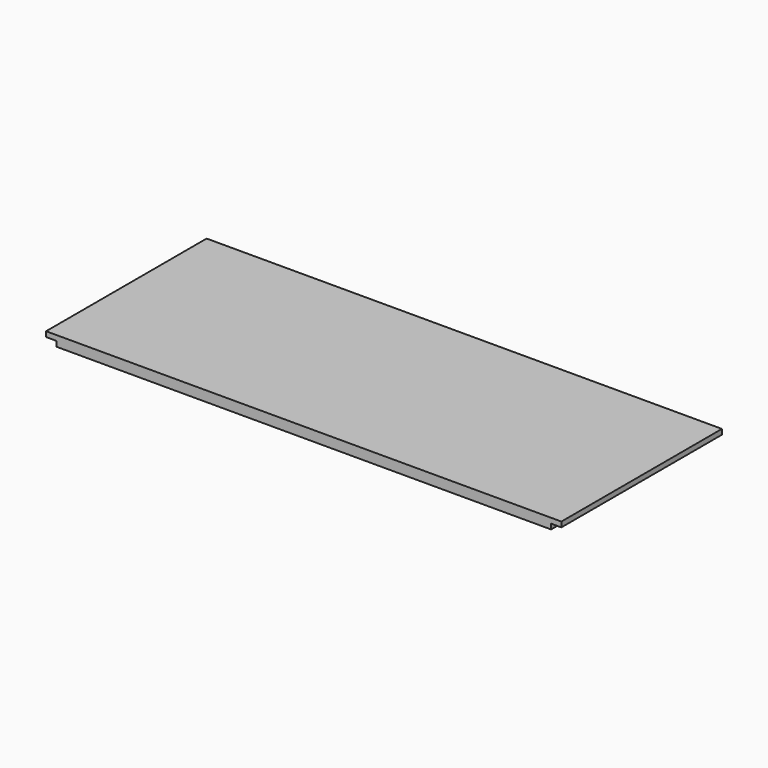
from build123d import *

# Parameters (mm, degrees)
F1_W      = 603.25
F1_H      = 234.95
F2_DEPTH  = 12.065
F3_W      = 12.065
F3_H      = 234.95
F4_DEPTH  = 6.0325
F5_W      = 12.065
F5_H      = 234.95
F6_DEPTH  = 6.0325
F7_W      = 12.065
F7_H      = 234.95
F8_DEPTH  = 6.0325
F9_W      = 12.065
F9_H      = 234.95
F10_DEPTH = 6.0325
F11_W     = 203.2
F11_H     = 12.065
F14_DEPTH = 6.0325
F12_W     = 148.59
F12_H     = 12.065
F15_DEPTH = 6.0325
F13_W     = 203.2
F13_H     = 12.065
F16_DEPTH = 6.0325
F17_W     = 12.065
F17_H     = 31.75
F18_DEPTH = 6.0325
F19_W     = 12.065
F19_H     = 31.75
F20_DEPTH = 6.0325


# Not quite as in the source:
# - a variable given as a bare number and used for a length is read in inches; the dataset says mm whatever the document's units were


with BuildPart() as f2:
    # F1 (on Top) → F2 (new body)
    with BuildSketch(Plane.XY):
        Rectangle(F1_W, F1_H)
    extrude(amount=F2_DEPTH)

    # F3 (on face) → F4 (cut)
    with BuildSketch(Plane(origin=(0, 0, 0), x_dir=(1, 0, 0), z_dir=(0, 0, -1))):
        with Locations((-295.5925, 0)):
            Rectangle(F3_W, F3_H)
    extrude(amount=-F4_DEPTH, mode=Mode.SUBTRACT)

    # F5 (on face) → F6 (cut)
    with BuildSketch(Plane(origin=(0, 0, 0), x_dir=(1, 0, 0), z_dir=(0, 0, -1))):
        with Locations((295.5925, 0)):
            Rectangle(F5_W, F5_H)
    extrude(amount=-F6_DEPTH, mode=Mode.SUBTRACT)

    # F7 (on face) → F8 (cut)
    with BuildSketch(Plane(origin=(0, 0, 0), x_dir=(1, 0, 0), z_dir=(0, 0, -1))):
        with Locations((80.3275, 0)):
            Rectangle(F7_W, F7_H)
    extrude(amount=-F8_DEPTH, mode=Mode.SUBTRACT)

    # F9 (on face) → F10 (cut)
    with BuildSketch(Plane(origin=(0, 0, 0), x_dir=(1, 0, 0), z_dir=(0, 0, -1))):
        with Locations((-80.3275, 0)):
            Rectangle(F9_W, F9_H)
    extrude(amount=-F10_DEPTH, mode=Mode.SUBTRACT)

    # F11 (on face) → F14 (cut)
    with BuildSketch(Plane(origin=(0, 0, 0), x_dir=(1, 0, 0), z_dir=(0, 0, -1))):
        with Locations((187.96, -111.4425)):
            Rectangle(F11_W, F11_H)
    extrude(amount=-F14_DEPTH, mode=Mode.SUBTRACT)

    # F12 (on face) → F15 (cut)
    with BuildSketch(Plane(origin=(0, 0, 0), x_dir=(1, 0, 0), z_dir=(0, 0, -1))):
        with Locations((0, -111.4425)):
            Rectangle(F12_W, F12_H)
    extrude(amount=-F15_DEPTH, mode=Mode.SUBTRACT)

    # F13 (on face) → F16 (cut)
    with BuildSketch(Plane(origin=(0, 0, 0), x_dir=(1, 0, 0), z_dir=(0, 0, -1))):
        with Locations((-187.96, -111.4425)):
            Rectangle(F13_W, F13_H)
    extrude(amount=-F16_DEPTH, mode=Mode.SUBTRACT)

    # F17 (on face) → F18 (join)
    with BuildSketch(Plane(origin=(0, 0, 6.0325), x_dir=(1, 0, 0), z_dir=(0, 0, -1))):
        with Locations((80.3275, 101.6)):
            Rectangle(F17_W, F17_H)
    extrude(amount=F18_DEPTH)

    # F19 (on face) → F20 (join)
    with BuildSketch(Plane(origin=(0, 0, 6.0325), x_dir=(1, 0, 0), z_dir=(0, 0, -1))):
        with Locations((-80.3275, 101.6)):
            Rectangle(F19_W, F19_H)
    extrude(amount=F20_DEPTH)


solid = f2.part
